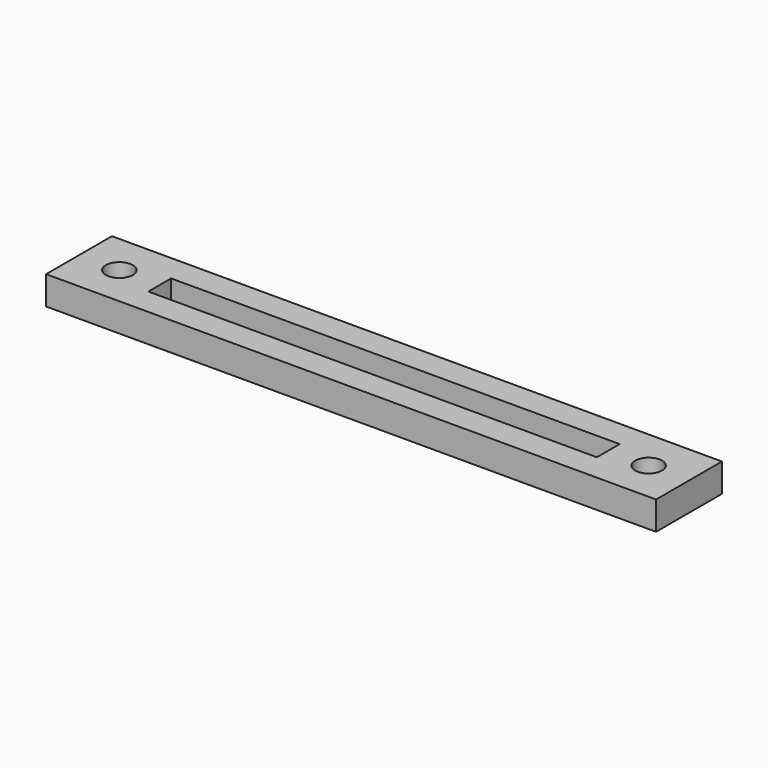
from build123d import *

# Parameters (mm, degrees)
F0_W     = 68
F0_H     = 9.175
F0_R     = 1.5
F1_DEPTH = 3.175


# Not quite as in the source:
# - a length typed as a fraction of an inch, garbled in the dataset ("3 / 203.2 mm" for 3/8 in), is restored


with BuildPart() as f1:
    # F0 (on Top) → F1 (new body)
    with BuildSketch(Plane.XY):
        with Locations((28.9220271409, 16.632870598)):
            Rectangle(F0_W, F0_H)
        with Locations((-0.5779728591, 16.632870598)):
            Circle(F0_R, mode=Mode.SUBTRACT)
        Polygon((3.9220271409, 15.045370598), (3.9220271409, 18.220370598), (28.9220271409, 18.220370598), (53.9220271409, 18.220370598), (53.9220271409, 15.045370598), align=None, mode=Mode.SUBTRACT)
        with Locations((58.4220271409, 16.632870598)):
            Circle(F0_R, mode=Mode.SUBTRACT)
    extrude(amount=F1_DEPTH)


solid = f1.part
